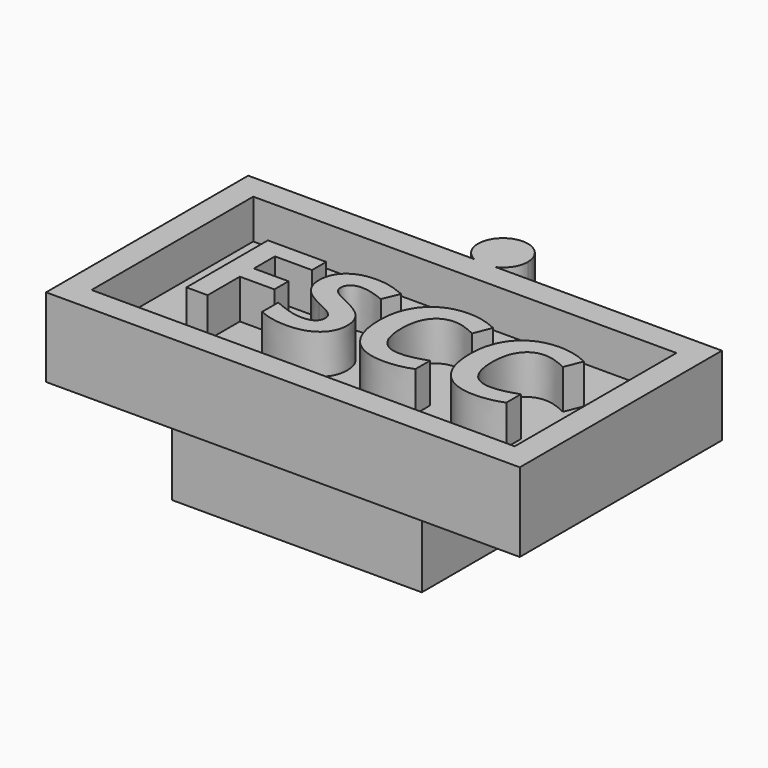
from build123d import *

# Parameters (mm, degrees)
F1_DEPTH     = 3.175
F2_W         = 17.018
F2_H         = 8.128
F3_DEPTH     = 1.5875
F4_W         = 10.05
F4_H         = 8.76
F5_DEPTH     = 3
F6_R         = 3.5
F7_DEPTH     = 3.5
F8_TEXT_SIZE = 5.7333333333
F9_DEPTH     = 1.5875


# Not quite as in the source:
# - Text() gives the source's letters only with a copy of the font that has no kerning and outlines rounded to 1/6400 em; it was checked with that copy


with BuildPart() as f1:
    # F0 (on Top) → F1 (new body)
    with BuildSketch(Plane.XY):
        with BuildLine():
            Line((-9.9608898944, 10.16), (-19.05, 10.16))
            Line((-19.05, 10.16), (-19.05, 0))
            Line((-19.05, 0), (0, 0))
            Line((0, 0), (0, 10.16))
            Line((0, 10.16), (-9.0891101056, 10.16))
            ThreePointArc((-9.0891101056, 10.16), (-9.525, 10.06), (-9.9608898944, 10.16))
        make_face()
        with BuildLine():
            ThreePointArc((-8.525, 11.06), (-10.0560885546, 11.9073163206), (-9.9608898944, 10.16))
            Line((-9.9608898944, 10.16), (-9.0891101056, 10.16))
            ThreePointArc((-9.0891101056, 10.16), (-8.6776836794, 10.5289114454), (-8.525, 11.06))
        make_face()
        with BuildLine():
            Line((-9.0891101056, 10.16), (-9.9608898944, 10.16))
            ThreePointArc((-9.9608898944, 10.16), (-9.525, 10.06), (-9.0891101056, 10.16))
        make_face()
    extrude(amount=F1_DEPTH)

    # F2 (on face) → F3 (cut)
    with BuildSketch(Plane.XY.offset(3.175)):
        with Locations((-9.525, 5.08)):
            Rectangle(F2_W, F2_H)
    extrude(amount=-F3_DEPTH, mode=Mode.SUBTRACT)

    # F4 (on face) → F5 (join)
    with BuildSketch(Plane(origin=(0, 0, 0), x_dir=(1, 0, 0), z_dir=(0, 0, -1))):
        with Locations((-9.525, -5.08)):
            Rectangle(F4_W, F4_H)
    extrude(amount=F5_DEPTH)

    # F6 (on face) → F7 (cut)
    with BuildSketch(Plane(origin=(0, 0, -3), x_dir=(1, 0, 0), z_dir=(0, 0, -1))):
        with Locations((-9.525, -5.08)):
            Circle(F6_R)
    extrude(amount=-F7_DEPTH, mode=Mode.SUBTRACT)

    # F8 (on face) → F9 (join, through all)
    with BuildSketch(Plane.XY.offset(1.5875)):
        with Locations((-16.334, 3.016)):
            Text('FSCC', F8_TEXT_SIZE, font='Open Sans', font_style=FontStyle.BOLD, text_align=(TextAlign.LEFT, TextAlign.BOTTOM))
    extrude(amount=F9_DEPTH)


solid = f1.part
